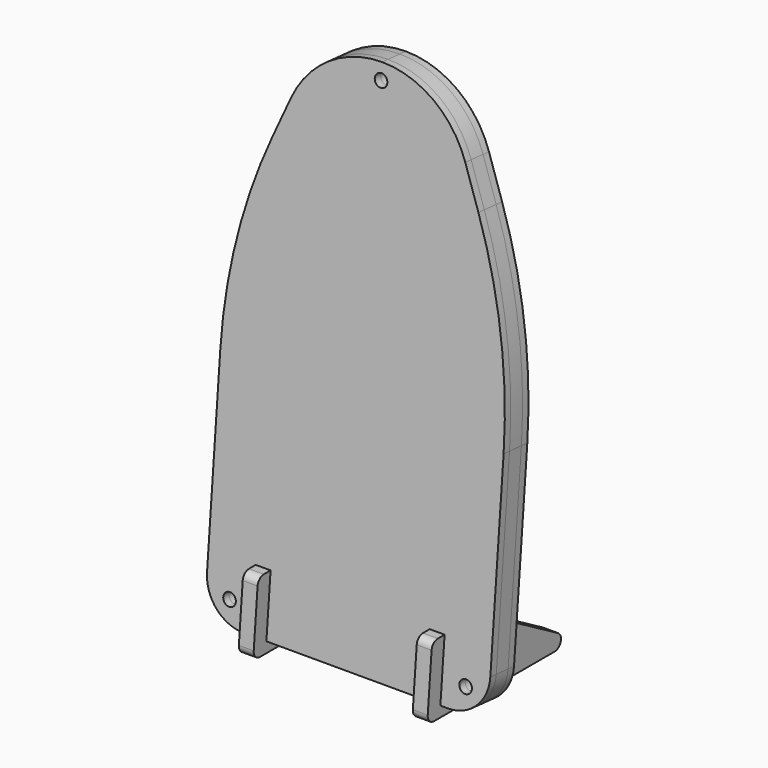
from build123d import *

# Parameters (mm, degrees)
F2_DEPTH  = 6
F4_W      = 6
F4_H      = 19.1227679052
F5_DEPTH  = 3
F6_R      = 203.2
F7_R      = 38.09999
F8_R      = 15.875
F9_DEPTH  = 6
F10_DEPTH = 3
F11_R     = 2.54
F12_DEPTH = 25.4


# Not quite as in the source:
# - a fillet or chamfer is up to 0.001 mm smaller than in the source, because OpenCascade refuses the exact size


with BuildPart() as f2:
    # F1 (on offset) → F2 (new body)
    with BuildSketch(Plane.YZ.offset(-38.1)):
        with BuildLine():
            ThreePointArc((0.3019863245, 3.4517194832), (1.1240489465, 1.0300010908), (3.4649044909, 0))
            Line((3.4649044909, 0), (64.350738686, 0))
            ThreePointArc((64.350738686, 0), (67.4175531844, 2.3532495318), (65.938238686, 5.924630657))
            Line((65.938238686, 5.924630657), (27.4434094878, 28.149630657))
            ThreePointArc((27.4434094878, 28.149630657), (26.677659956, 28.4668144985), (25.8559094878, 28.575))
            Line((25.8559094878, 28.575), (20.8499885603, 28.575))
            Line((20.8499885603, 28.575), (19.1833295201, 9.525))
            Line((19.1833295201, 9.525), (7.1833295201, 9.525))
            Line((7.1833295201, 9.525), (8.8499885603, 28.575))
            Line((8.8499885603, 28.575), (5.4093400378, 28.575))
            ThreePointArc((5.4093400378, 28.575), (3.2643411286, 27.7408555444), (2.2464218713, 25.6767194832))
            Line((2.2464218713, 25.6767194832), (0.3019863245, 3.4517194832))
        make_face()
    extrude(amount=F2_DEPTH)


with BuildPart() as f3_1:
    # F3: instance of F2
    add(f2.part.mirror(Plane.YZ))


with BuildPart() as f5:
    # F4 (on face) → F5 (new body)
    with BuildSketch(Plane(origin=(0, 18.2106111339, -1.5932220301), x_dir=(1, 0, 0), z_dir=(0, -0.9961946981, 0.0871557427))):
        Polygon((32.1, 11.160691832), (38.1, 11.160691832), (38.1, 4.810691832), (57.15, 4.810691832), (57.15, 11.160691832), (57.15, 138.160691832), (25.4, 214.360691832), (-25.4, 214.360691832), (-57.15, 138.160691832), (-57.15, 11.160691832), (-57.15, 4.810691832), (-38.1, 4.810691832), (-38.1, 11.160691832), (-38.1, 30.2834597372), (-32.1, 30.2834597372), (-32.1, 11.160691832), (-32.1, 4.810691832), (32.1, 4.810691832), align=None)
        with Locations((-35.1, 20.7220757846)):
            Rectangle(F4_W, F4_H)
    extrude(amount=F5_DEPTH)

    # F6
    f6_edges = [f5.edges().sort_by_distance(p)[0] for p in [
        (-57.15, 28.757817, 136.17246),
        (57.15, 28.757817, 136.17246),
    ]]
    fillet(f6_edges, radius=F6_R)

    # F7 (radius 38.1 in the source; OpenCascade refuses exactly that, so slightly less here)
    f7_edges = [f5.edges().sort_by_distance(p)[0] for p in [
        (-25.4, 35.399084, 212.082496),
        (25.4, 35.399084, 212.082496),
    ]]
    fillet(f7_edges, radius=F7_R)

    # F8
    f8_edges = [f5.edges().sort_by_distance(p)[0] for p in [
        (-57.15, 17.135599, 3.329897),
        (57.15, 17.135599, 3.329897),
    ]]
    fillet(f8_edges, radius=F8_R)


with BuildPart() as f9:
    # F9 (new): a face of the model
    f9_faces = [f5.part.faces().sort_by_distance(p)[0] for p in [
        (0, 23.9302542283, 98.2037374296),
    ]]
    extrude(f9_faces, amount=F9_DEPTH)


with BuildPart() as f10:
    # F10 (new): a face of the model
    f10_faces = [f9.part.faces().sort_by_distance(p)[0] for p in [
        (0, 17.9530860398, 98.7266718861),
    ]]
    extrude(f10_faces, amount=F10_DEPTH)


with BuildPart() as f12_tool:
    # F11 (on face) → F12 (new body)
    with BuildSketch(Plane(origin=(0, 6.2562747568, -0.5473531171), x_dir=(1, 0, 0), z_dir=(0, -0.9961946981, 0.0871557427))):
        with Locations((-47.625, 14.335691832)):
            Circle(F11_R)
        with Locations((47.625, 14.335691832)):
            Circle(F11_R)
        with Locations((0, 208.010691832)):
            Circle(F11_R)
    extrude(amount=-F12_DEPTH)


with BuildPart() as f5_1:
    add(f5.part)

    # F12: cut by f12_tool
    add(f12_tool.part, mode=Mode.SUBTRACT)


with BuildPart() as f9_1:
    add(f9.part)

    # F12: cut by f12_tool
    add(f12_tool.part, mode=Mode.SUBTRACT)


with BuildPart() as f10_1:
    add(f10.part)

    # F12: cut by f12_tool
    add(f12_tool.part, mode=Mode.SUBTRACT)


solid = Compound([f2.part, f3_1.part, f5_1.part, f9_1.part, f10_1.part])
